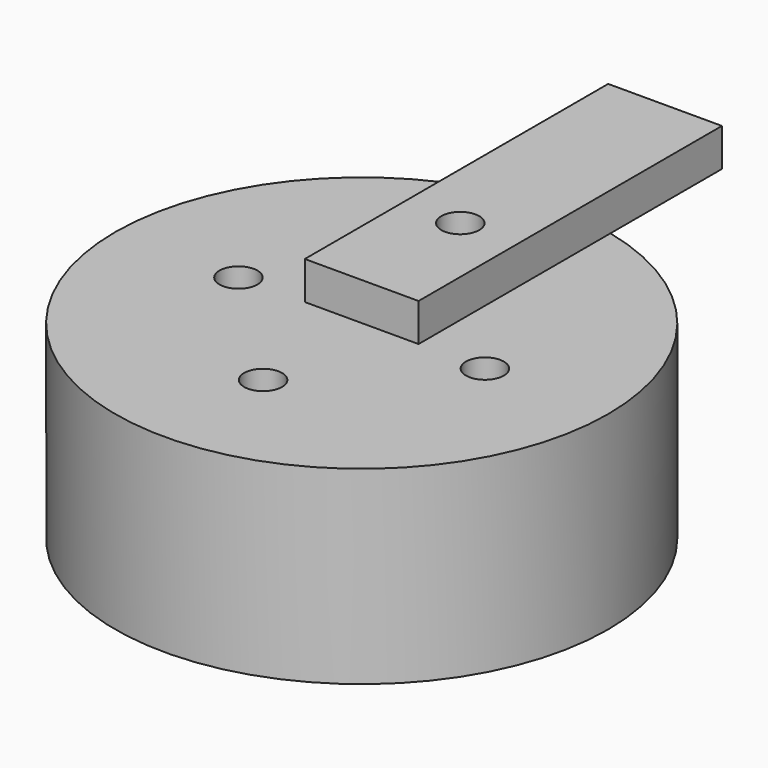
from build123d import *

# Parameters (mm, degrees)
F0_R            = 6.5
F1_DEPTH        = 5
F2_R            = 0.5
F3_DEPTH        = 2
F3_COPIES_COUNT = 4
F4_R            = 0.5
F5_DEPTH        = 1


# Not quite as in the source:
# - a pattern or mirror of a feature is missing from the dataset's text; its kind, count and spacing are read off the source's solid


with BuildPart() as f1:
    # F0 (on Top) → F1 (new body)
    with BuildSketch(Plane.XY):
        Circle(F0_R)
    extrude(amount=F1_DEPTH)

    # F2 (on face) → F3 (cut)
    with BuildSketch(Plane.XY.offset(5)):
        with Locations((0, 3.25)):
            Circle(F2_R)
    f3 = extrude(amount=-F3_DEPTH, mode=Mode.SUBTRACT)

    # F3_copies: F3 ×4 about axis
    f3_copies_axis = Axis((0, 0, 0), (0, 0, 1))
    for i in range(1, F3_COPIES_COUNT):
        add(f3.rotate(f3_copies_axis, i * 360 / F3_COPIES_COUNT), mode=Mode.SUBTRACT)

    # F4 (on face) → F5 (join)
    with BuildSketch(Plane.XY.offset(5)):
        with BuildLine():
            Line((-1.5, 10), (-1.5, 6.3245553203))
            ThreePointArc((-1.5, 6.3245553203), (0, 6.5), (1.5, 6.3245553203))
            Line((1.5, 6.3245553203), (1.5, 10))
            Line((1.5, 10), (-1.5, 10))
        make_face()
        with BuildLine():
            Line((-1.5, 6.3245553203), (-1.5, 0))
            Line((-1.5, 0), (1.5, 0))
            Line((1.5, 0), (1.5, 6.3245553203))
            ThreePointArc((1.5, 6.3245553203), (0, 6.5), (-1.5, 6.3245553203))
        make_face()
        with Locations((0, 3.25)):
            Circle(F4_R, mode=Mode.SUBTRACT)
    extrude(amount=F5_DEPTH)


solid = f1.part
